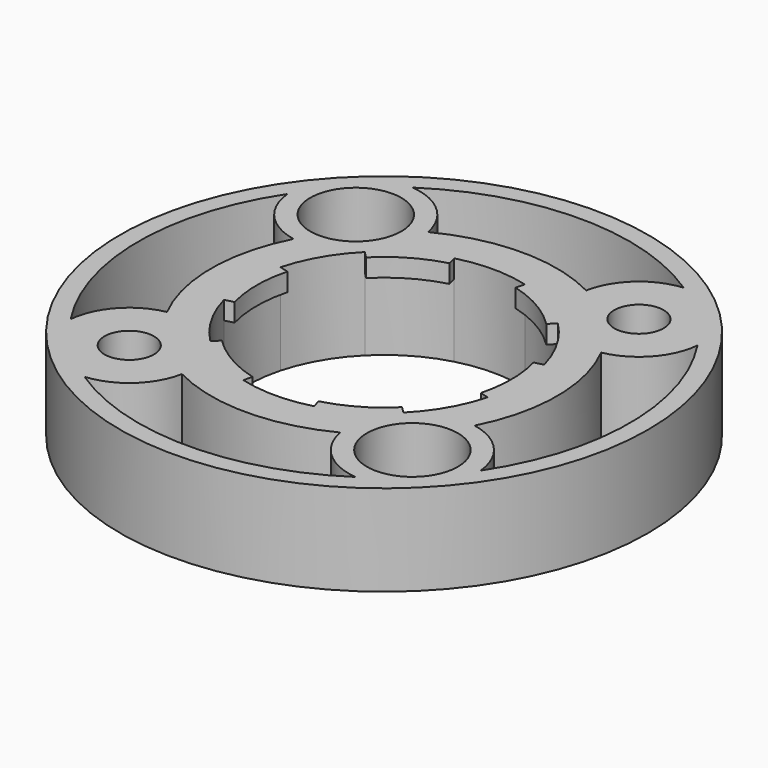
from build123d import *

# Parameters (mm, degrees)
F0_R            = 23.01875
F0_R_2          = 2.15265
F0_R_3          = 3.96875
F0_R_4          = 11.1125
F1_DEPTH        = 7.9375
F3_DEPTH        = 7.9375
F4_COUNT        = 6
F4_ANGLE        = 300
F6_R            = 11.90625
F7_DEPTH        = 6.35
F9_DEPTH        = 7.9375
F9_COPIES_COUNT = 4


# Not quite as in the source:
# - a pattern or mirror of a feature is missing from the dataset's text; its kind, count and spacing are read off the source's solid


with BuildPart() as f1:
    # F0 (on Top) → F1 (new body)
    with BuildSketch(Plane.XY):
        Circle(F0_R)
        with Locations((-12.3478521665, -12.3478521665)):
            Circle(F0_R_2, mode=Mode.SUBTRACT)
        with Locations((12.3478521665, -12.3478521665)):
            Circle(F0_R_3, mode=Mode.SUBTRACT)
        with Locations((-12.3478521665, 12.3478521665)):
            Circle(F0_R_3, mode=Mode.SUBTRACT)
        Circle(F0_R_4, mode=Mode.SUBTRACT)
        with Locations((12.3478521665, 12.3478521665)):
            Circle(F0_R_2, mode=Mode.SUBTRACT)
    extrude(amount=F1_DEPTH)

    # F2 (on face) → F3 (cut, through all)
    with BuildSketch(Plane.XY.offset(7.9375)):
        with BuildLine():
            Line((-3.0815642558, 11.5005543693), (-2.8761266387, 10.7338507446))
            ThreePointArc((-2.8761266387, 10.7338507446), (0, 11.1125), (2.8761266387, 10.7338507446))
            Line((2.8761266387, 10.7338507446), (3.0815642558, 11.5005543693))
            ThreePointArc((3.0815642558, 11.5005543693), (0, 11.90625), (-3.0815642558, 11.5005543693))
        make_face()
    f3 = extrude(amount=-F3_DEPTH, mode=Mode.SUBTRACT)

    # F4: F3 ×6 about axis
    f4_axis = Axis((0, 0, 0), (0, 0, -1))
    for i in range(1, F4_COUNT):
        add(f3.rotate(f4_axis, i * F4_ANGLE / (F4_COUNT - 1)), mode=Mode.SUBTRACT)

    # F6 (on face) → F7 (cut, through all)
    with BuildSketch(Plane(origin=(0, 0, 0), x_dir=(1, 0, 0), z_dir=(0, 0, -1))):
        Circle(F6_R)
    extrude(amount=-F7_DEPTH, mode=Mode.SUBTRACT)

    # F8 (on face) → F9 (cut, through all)
    with BuildSketch(Plane(origin=(0, 0, 0), x_dir=(1, 0, 0), z_dir=(0, 0, -1))):
        with BuildLine():
            ThreePointArc((-13.4129757356, 6.8946489019), (-16.4630716815, 8.614638751), (-17.8787189274, 11.8173552911))
            ThreePointArc((-17.8787189274, 11.8173552911), (-21.43125, 0), (-17.8787189274, -11.8173552911))
            ThreePointArc((-17.8787189274, -11.8173552911), (-16.4630716815, -8.614638751), (-13.4129757356, -6.8946489019))
            ThreePointArc((-13.4129757356, -6.8946489019), (-15.08125, 0), (-13.4129757356, 6.8946489019))
        make_face()
    f9 = extrude(amount=-F9_DEPTH, mode=Mode.SUBTRACT)

    # F9_copies: F9 ×4 about axis
    f9_copies_axis = Axis((0, 0, 0), (0, 0, 1))
    for i in range(1, F9_COPIES_COUNT):
        add(f9.rotate(f9_copies_axis, i * 360 / F9_COPIES_COUNT), mode=Mode.SUBTRACT)


solid = f1.part
